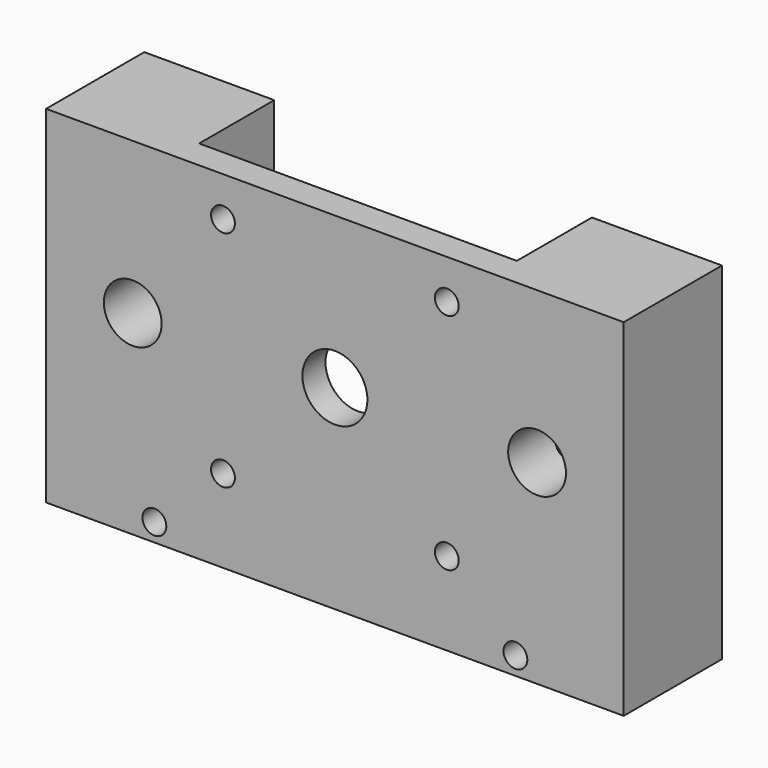
from build123d import *

# Parameters (mm, degrees)
F0_W      = 80
F0_H      = 17
F0_R      = 1.05
F1_DEPTH  = 2.5
F3_DEPTH  = 43
F5_DEPTH  = 25
F7_D      = 3.3
F8_D      = 3.3
F4_R      = 4.5
F9_DEPTH  = 4.0010001
F10_R     = 4
F11_DEPTH = 10


# Not quite as in the source:
# - a feature names something its author has since deleted; it is built from what else it names


with BuildPart() as f1:
    # F0 (on Top) → F1 (new body, symmetric)
    with BuildSketch(Plane.XY):
        Rectangle(F0_W, F0_H)
        with Locations((-25, 0)):
            Circle(F0_R, mode=Mode.SUBTRACT)
        Circle(F0_R, mode=Mode.SUBTRACT)
        with Locations((25, 0)):
            Circle(F0_R, mode=Mode.SUBTRACT)
    extrude(amount=F1_DEPTH, both=True)

    # F2 (on face) → F3 (join)
    with BuildSketch(Plane.XY.offset(2.5)):
        Polygon((-40, -8.5), (40, -8.5), (40, 8.5), (22, 8.5), (22, -4.5), (-22, -4.5), (-22, 8.5), (-40, 8.5), align=None)
    extrude(amount=F3_DEPTH)

    # F0 (on Top) → F5 (cut)
    with BuildSketch(Plane.XY):
        with Locations((-25, 0)):
            Circle(F0_R)
        Circle(F0_R)
        with Locations((25, 0)):
            Circle(F0_R)
    extrude(amount=F5_DEPTH, mode=Mode.SUBTRACT)

    # F7 (through all)
    with Locations(Plane(origin=(0, 8.5, 0), x_dir=(-1, 0, 0), z_dir=(0, 1, 0))):
        with Locations((25, 0), (-25, 0)):
            Hole(F7_D / 2)

    # F8 (through all)
    with Locations(Plane(origin=(0, -4.5, 0), x_dir=(-1, 0, 0), z_dir=(0, 1, 0))):
        with Locations((15.5, 40), (-15.5, 40), (-15.5, 9), (15.5, 9)):
            Hole(F8_D / 2)

    # F4 (on face) → F9 (cut, through all)
    with BuildSketch(Plane(origin=(0, -4.5, 0), x_dir=(-1, 0, 0), z_dir=(0, 1, 0))):
        with Locations((0, 24.5)):
            Circle(F4_R)
    extrude(amount=-F9_DEPTH, mode=Mode.SUBTRACT)

    # F10 (on face) → F11 (cut)
    with BuildSketch(Plane.XZ.offset(8.5)):
        with Locations((-28, 24.5)):
            Circle(F10_R)
        with Locations((28, 24.5)):
            Circle(F10_R)
    extrude(amount=-F11_DEPTH, mode=Mode.SUBTRACT)


solid = f1.part
